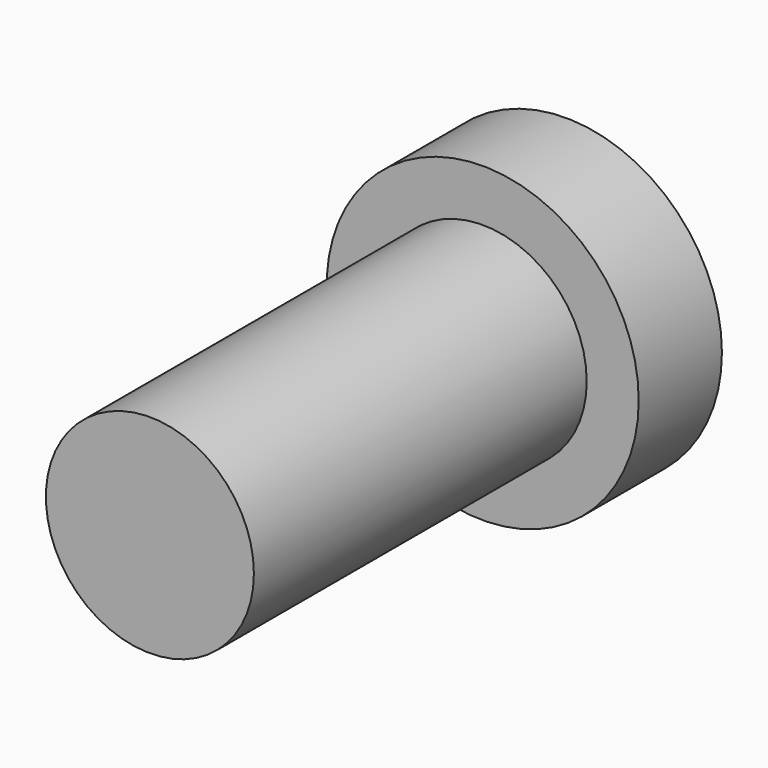
from build123d import *

# Parameters (mm, degrees)
F0_R     = 10
F1_DEPTH = 40
F0_R_2   = 15
F2_DEPTH = 10


# Not quite as in the source:
# - a feature names something its author has since deleted; it is built from what else it names


with BuildPart() as f1:
    # F0 (on Front) → F1 (new body)
    with BuildSketch(Plane.XZ):
        Circle(F0_R)
    extrude(amount=F1_DEPTH)

    # F0 (on Front) → F2 (join)
    with BuildSketch(Plane.XZ):
        Circle(F0_R_2)
        Circle(F0_R, mode=Mode.SUBTRACT)
        Circle(F0_R)
    extrude(amount=-F2_DEPTH)


solid = f1.part
